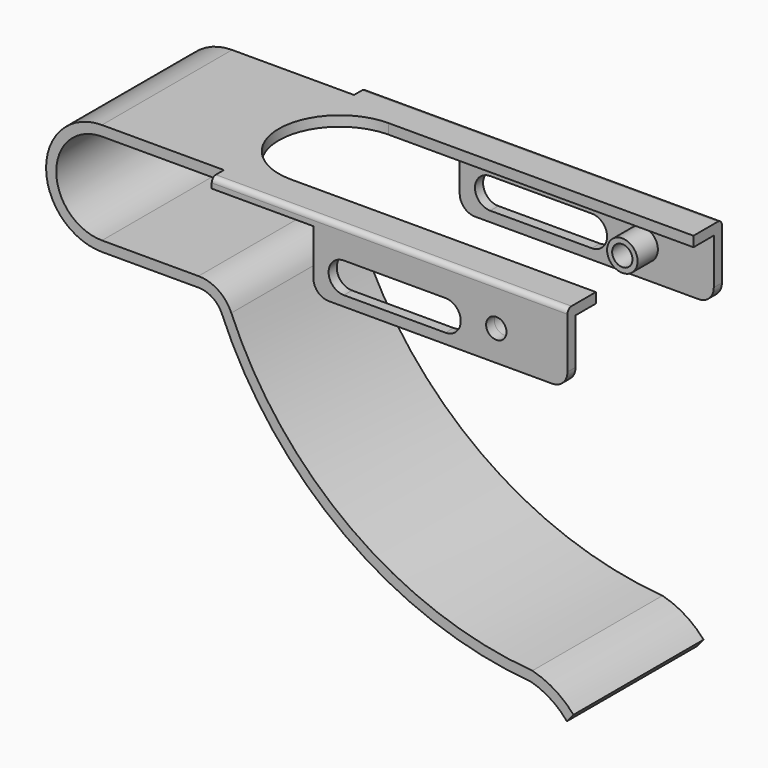
from build123d import *

# Parameters (mm, degrees)
F1_DEPTH  = 16
F2_W      = 70
F2_H      = 3
F3_DEPTH  = 2
F4_W      = 50
F4_H      = 12
F5_DEPTH  = 2
F6_R      = 1
F9_DEPTH  = 2
F11_DEPTH = 38.001
F13_D     = 4
F14_R     = 3
F14_R_2   = 2
F15_DEPTH = 5
F16_R     = 3


# Not quite as in the source:
# - a pattern or mirror of a feature is missing from the dataset's text; its kind, count and spacing are read off the source's solid


with BuildPart() as f1:
    # F0 (on Front) → F1 (new body)
    with BuildSketch(Plane.XZ):
        with BuildLine():
            Line((94, 11), (0, 11))
            ThreePointArc((0, 11), (-11, 0), (0, -11))
            Line((0, -11), (19, -11))
            ThreePointArc((19, -11), (21.7681124643, -11.8361612201), (23.6103896104, -14.064978646))
            ThreePointArc((23.6103896104, -14.064978646), (47.8232093534, -44.5540629158), (84.3688749643, -57.9801280344))
            ThreePointArc((84.3688749643, -57.9801280344), (88.282737688, -59.7162176184), (91.4888593469, -62.5540182408))
            Line((91.4888593469, -62.5540182408), (92.7928354795, -61))
            ThreePointArc((92.7928354795, -61), (89.1281978331, -57.8850966861), (84.7034264019, -56))
            ThreePointArc((84.7034264019, -56), (49.0672193413, -42.9854179344), (25.4545454545, -13.2909701044))
            ThreePointArc((25.4545454545, -13.2909701044), (22.87535745, -10.1706257081), (19, -9))
            Line((19, -9), (0, -9))
            ThreePointArc((0, -9), (-9, 0), (0, 9))
            Line((0, 9), (94, 9))
            Line((94, 9), (94, 11))
        make_face()
    extrude(amount=F1_DEPTH)

    # F2 (on face) → F3 (join)
    with BuildSketch(Plane.XY.offset(11)):
        with Locations((59, -17.5)):
            Rectangle(F2_W, F2_H)
    extrude(amount=-F3_DEPTH)

    # F4 (on face) → F5 (join)
    with BuildSketch(Plane.XZ.offset(19)):
        with Locations((69, 3)):
            Rectangle(F4_W, F4_H)
    extrude(amount=-F5_DEPTH)

    # F6
    f6_edges = [f1.edges().sort_by_distance(p)[0] for p in [
        (59, -19, 11),
    ]]
    fillet(f6_edges, radius=F6_R)

    # F7: F1 across plane


with BuildPart() as f1_1:
    add(f1.part)
    add(f1.part.mirror(Plane.XZ))

    # F8 (on face) → F9 (cut)
    with BuildSketch(Plane.XY.offset(11)):
        with BuildLine():
            Line((94, 12), (34, 12))
            ThreePointArc((34, 12), (22, 0), (34, -12))
            Line((34, -12), (94, -12))
            Line((94, -12), (94, 12))
        make_face()
    extrude(amount=-F9_DEPTH, mode=Mode.SUBTRACT)

    # F10 (on face) → F11 (cut, through all)
    with BuildSketch(Plane.XZ.offset(19)):
        with BuildLine():
            ThreePointArc((50, 5), (47, 2), (50, -1))
            Line((50, -1), (70, -1))
            ThreePointArc((70, -1), (73, 2), (70, 5))
            Line((70, 5), (50, 5))
        make_face()
    extrude(amount=-F11_DEPTH, mode=Mode.SUBTRACT)

    # F13 (through all)
    with Locations(Plane.XZ.offset(19)):
        with Locations((80, 3)):
            Hole(F13_D / 2)

    # F14 (on face) → F15 (join)
    with BuildSketch(Plane(origin=(0, -17, 0), x_dir=(-1, 0, 0), z_dir=(0, 1, 0))):
        with Locations((-80, 3)):
            Circle(F14_R)
        with Locations((-80, 3)):
            Circle(F14_R_2, mode=Mode.SUBTRACT)
    f15 = extrude(amount=F15_DEPTH)

    # F15_copies: F15 across plane
    add(f15.mirror(Plane.ZX))

    # F16
    f16_edges = [f1_1.edges().sort_by_distance(p)[0] for p in [
        (94, 18, -3),
        (44, 18, -3),
        (94, -18, -3),
        (44, -18, -3),
    ]]
    fillet(f16_edges, radius=F16_R)


solid = f1_1.part
